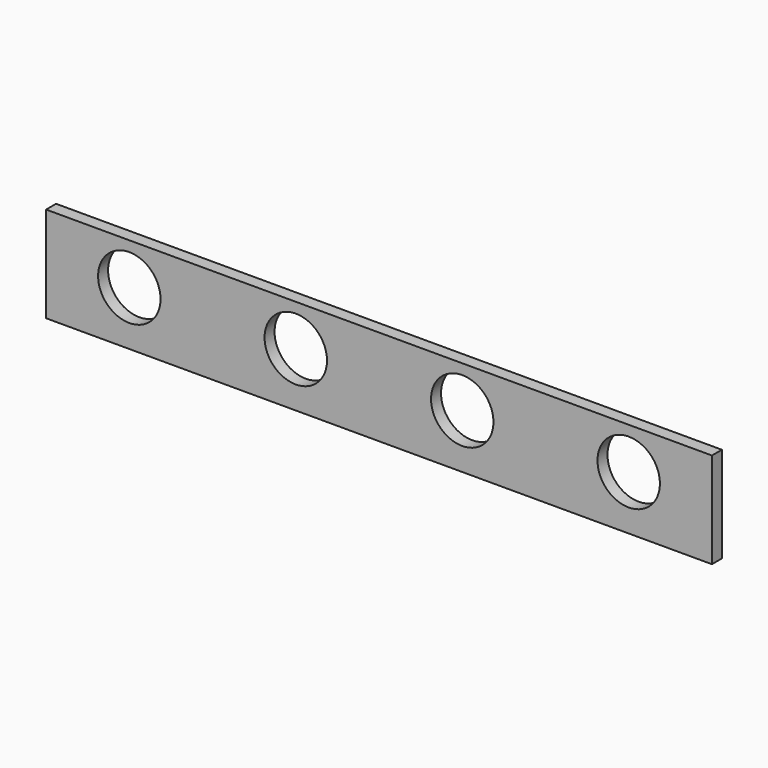
from build123d import *

# Parameters (mm, degrees)
F0_W     = 1016
F0_H     = 146.05
F1_DEPTH = 19.05
F2_R     = 47.625
F3_DEPTH = 19.051


# Not quite as in the source:
# - a feature names something its author has since deleted; it is built from what else it names


with BuildPart() as f1:
    # F0 (on Front) → F1 (new body)
    with BuildSketch(Plane.XZ):
        with Locations((508, -73.025)):
            Rectangle(F0_W, F0_H)
    extrude(amount=F1_DEPTH)

    # F2 (on face) → F3 (cut, through all)
    with BuildSketch(Plane.XZ.offset(19.05)):
        with Locations((127, -63.5)):
            Circle(F2_R)
        with Locations((381, -63.5)):
            Circle(F2_R)
        with Locations((635, -63.5)):
            Circle(F2_R)
        with Locations((889, -63.5)):
            Circle(F2_R)
    extrude(amount=-F3_DEPTH, mode=Mode.SUBTRACT)


solid = f1.part
